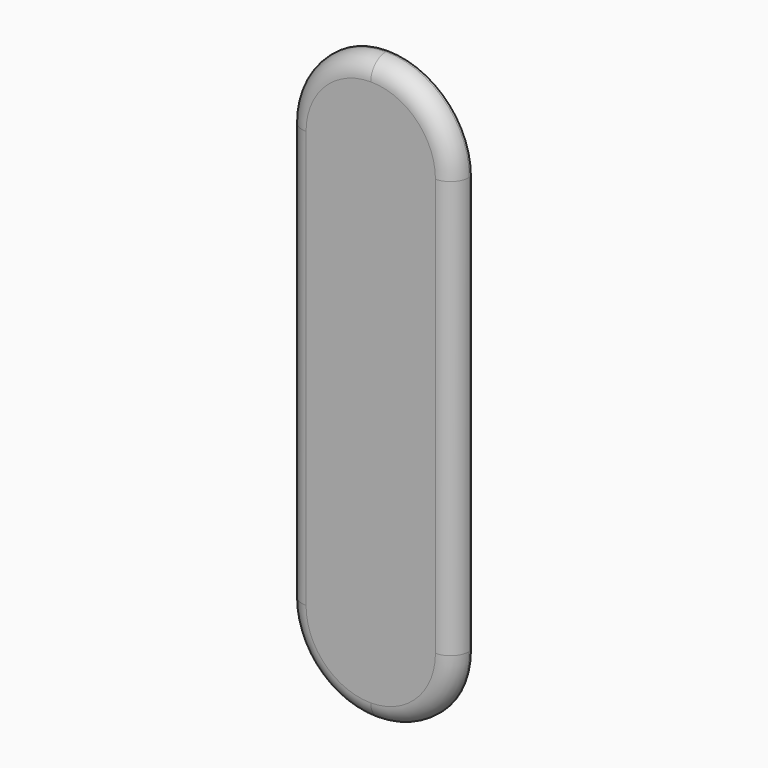
from build123d import *

# Parameters (mm, degrees)
F0_W      = 40
F0_H      = 140
F1_DEPTH  = 5
F2_R      = 19.99999
F3_R      = 4.5
F5_DEPTH  = 5
F6_W      = 12
F6_H      = 12
F7_DEPTH  = 3
F8_R      = 2
F10_DEPTH = 5


# Not quite as in the source:
# - a fillet or chamfer is up to 0.001 mm smaller than in the source, because OpenCascade refuses the exact size
# - a pattern or mirror of a feature is missing from the dataset's text; its kind, count and spacing are read off the source's solid


with BuildPart() as f1:
    # F0 (on Front) → F1 (new body)
    with BuildSketch(Plane.XZ):
        Rectangle(F0_W, F0_H)
    extrude(amount=F1_DEPTH)

    # F2 (radius 20 in the source; OpenCascade refuses exactly that, so slightly less here)
    f2_edges = [f1.edges().sort_by_distance(p)[0] for p in [
        (-20, -2.5, 70),
        (20, -2.5, 70),
        (20, -2.5, -70),
        (-20, -2.5, -70),
    ]]
    fillet(f2_edges, radius=F2_R)

    # F3
    f3_edges = [f1.edges().sort_by_distance(p)[0] for p in [
        (20, -5, 0),
        (0, -5, -70),
        (-14.142139, -5, -64.142139),
        (14.142139, -5, -64.142139),
        (-20, -5, 0),
        (-14.142139, -5, 64.142139),
        (14.142139, -5, 64.142139),
        (0, -5, 70),
    ]]
    fillet(f3_edges, radius=F3_R)

    # F4 (on face) → F5 (join)
    with BuildSketch(Plane(origin=(0, 0, 0), x_dir=(-1, 0, 0), z_dir=(0, 1, 0))):
        with BuildLine():
            ThreePointArc((2.5399159699, 60.1534954225), (2.8826851987, 60.9192617469), (3, 61.75))
            ThreePointArc((3, 61.75), (2.9811636084, 62.0856538989), (2.9248909734, 62.4170927923))
            ThreePointArc((2.9248909734, 62.4170927923), (2.4469615912, 63.48562063), (1.5965045374, 64.2899159951))
            ThreePointArc((1.5965045374, 64.2899159951), (0.5029940174, 64.7075322515), (-0.6670927923, 64.6748909734))
            ThreePointArc((-0.6670927923, 64.6748909734), (-1.7356206048, 64.1969616091), (-2.5399159621, 63.3465045899))
            ThreePointArc((-2.5399159621, 63.3465045899), (-2.9575322502, 62.2529940246), (-2.9248909629, 61.0829071616))
            ThreePointArc((-2.9248909629, 61.0829071616), (-2.4469615928, 60.0143793723), (-1.5965045824, 59.2100840332))
            ThreePointArc((-1.5965045824, 59.2100840332), (-0.5029939825, 58.7924677426), (0.6670929131, 58.8251090541))
            ThreePointArc((0.6670929131, 58.8251090541), (1.7356206613, 59.303038431), (2.5399159699, 60.1534954225))
        make_face()
        with BuildLine():
            ThreePointArc((2.9248909734, 62.4170927923), (2.9811636084, 62.0856538989), (3, 61.75))
            ThreePointArc((3, 61.75), (2.8826851987, 60.9192617469), (2.5399159699, 60.1534954225))
            Line((2.5399159699, 60.1534954225), (3.2012098578, 61.2055632972))
            Line((3.2012098578, 61.2055632972), (2.9248909734, 62.4170927923))
        make_face()
        with BuildLine():
            ThreePointArc((1.5965045374, 64.2899159951), (2.4469615912, 63.48562063), (2.9248909734, 62.4170927923))
            Line((2.9248909734, 62.4170927923), (2.648572083, 63.628622314))
            Line((2.648572083, 63.628622314), (1.5965045374, 64.2899159951))
        make_face()
        with BuildLine():
            Line((1.878622314, 59.101427917), (2.5399159699, 60.1534954225))
            ThreePointArc((2.5399159699, 60.1534954225), (1.7356206613, 59.303038431), (0.6670929131, 58.8251090541))
            Line((0.6670929131, 58.8251090541), (1.878622314, 59.101427917))
        make_face()
        with BuildLine():
            ThreePointArc((-0.6670927923, 64.6748909734), (0.5029940174, 64.7075322515), (1.5965045374, 64.2899159951))
            Line((1.5965045374, 64.2899159951), (0.5444367028, 64.9512098578))
            Line((0.5444367028, 64.9512098578), (-0.6670927923, 64.6748909734))
        make_face()
        with BuildLine():
            Line((-0.5444367028, 58.5487901422), (0.6670929131, 58.8251090541))
            ThreePointArc((0.6670929131, 58.8251090541), (-0.5029939825, 58.7924677426), (-1.5965045824, 59.2100840332))
            Line((-1.5965045824, 59.2100840332), (-0.5444367028, 58.5487901422))
        make_face()
        with BuildLine():
            ThreePointArc((-2.5399159621, 63.3465045899), (-1.7356206048, 64.1969616091), (-0.6670927923, 64.6748909734))
            Line((-0.6670927923, 64.6748909734), (-1.878622314, 64.398572083))
            Line((-1.878622314, 64.398572083), (-2.5399159621, 63.3465045899))
        make_face()
        with BuildLine():
            Line((-2.648572083, 59.871377686), (-1.5965045824, 59.2100840332))
            ThreePointArc((-1.5965045824, 59.2100840332), (-2.4469615928, 60.0143793723), (-2.9248909629, 61.0829071616))
            Line((-2.9248909629, 61.0829071616), (-2.648572083, 59.871377686))
        make_face()
        with BuildLine():
            ThreePointArc((-2.9248909629, 61.0829071616), (-2.9575322502, 62.2529940246), (-2.5399159621, 63.3465045899))
            Line((-2.5399159621, 63.3465045899), (-3.2012098578, 62.2944367028))
            Line((-3.2012098578, 62.2944367028), (-2.9248909629, 61.0829071616))
        make_face()
    f5 = extrude(amount=F5_DEPTH)

    # F5_copies: F5 across plane
    add(f5.mirror(Plane(origin=(0, 0, 0), x_dir=(-1, 0, 0), z_dir=(0, 0, -1))))

    # F6 (on face) → F7 (cut)
    with BuildSketch(Plane(origin=(0, 0, 0), x_dir=(-1, 0, 0), z_dir=(0, 1, 0))):
        with Locations((0, 25.5)):
            Rectangle(F6_W, F6_H)
    f7 = extrude(amount=-F7_DEPTH, mode=Mode.SUBTRACT)

    # F7_copies: F7 across plane
    add(f7.mirror(Plane(origin=(0, 0, 0), x_dir=(-1, 0, 0), z_dir=(0, 0, -1))), mode=Mode.SUBTRACT)

    # F8
    f8_edges = [f1.edges().sort_by_distance(p)[0] for p in [
        (6, -1.5, 31.5),
        (-6, -1.5, 31.5),
        (-6, -1.5, 19.5),
        (6, -1.5, 19.5),
        (6, -1.5, -19.5),
        (-6, -1.5, -19.5),
        (-6, -1.5, -31.5),
        (6, -1.5, -31.5),
    ]]
    fillet(f8_edges, radius=F8_R)

    # F9 (on face) → F10 (join)
    with BuildSketch(Plane(origin=(0, 0, 0), x_dir=(-1, 0, 0), z_dir=(0, 1, 0))):
        with BuildLine():
            ThreePointArc((0, -41), (11.1369318037, -36.3869318037), (15.75, -25.25))
            Line((15.75, -25.25), (15.75, 25.25))
            ThreePointArc((15.75, 25.25), (11.1369318037, 36.3869318037), (0, 41))
            ThreePointArc((0, 41), (-11.1369318037, 36.3869318037), (-15.75, 25.25))
            Line((-15.75, 25.25), (-15.75, -25.25))
            ThreePointArc((-15.75, -25.25), (-11.1369318037, -36.3869318037), (0, -41))
        make_face()
        with BuildLine():
            ThreePointArc((12.75, -25.25), (9.0156114601, -34.2656114601), (0, -38))
            ThreePointArc((0, -38), (-9.0156114601, -34.2656114601), (-12.75, -25.25))
            Line((-12.75, -25.25), (-12.75, 25.25))
            ThreePointArc((-12.75, 25.25), (-9.0156114601, 34.2656114601), (0, 38))
            ThreePointArc((0, 38), (9.0156114601, 34.2656114601), (12.75, 25.25))
            Line((12.75, 25.25), (12.75, -25.25))
        make_face(mode=Mode.SUBTRACT)
    extrude(amount=F10_DEPTH)


solid = f1.part
